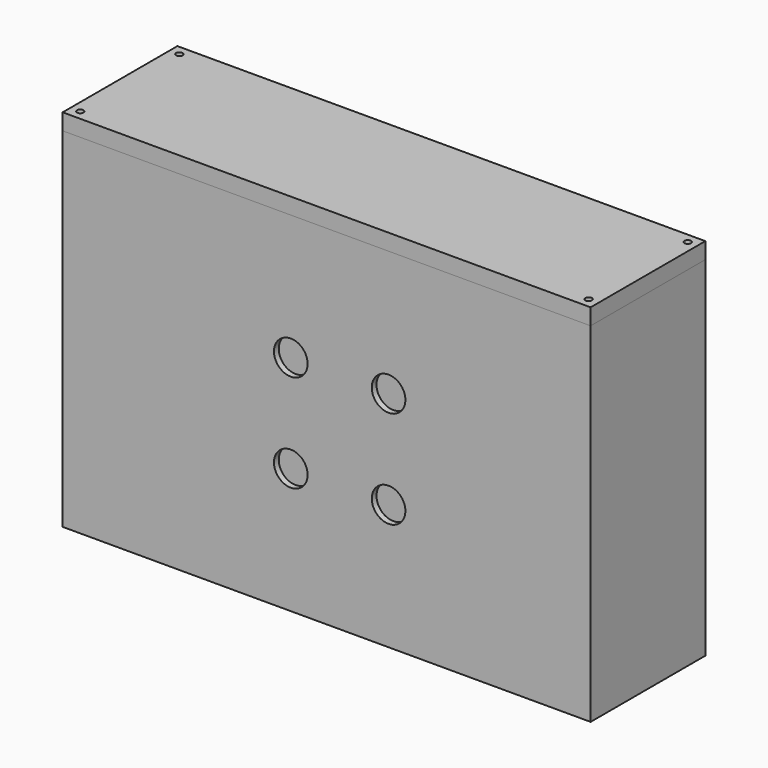
from build123d import *

# Parameters (mm, degrees)
F0_W      = 81
F0_H      = 53.5
F1_DEPTH  = 11
F2_T      = -2.5
F3_W      = 14
F3_H      = 5
F4_DEPTH  = 49.6
F5_R      = 2.5796875
F6_DEPTH  = 25
F8_W      = 81
F8_H      = 22
F9_DEPTH  = 2.5
F11_R     = 0.5
F12_DEPTH = 5
F10_R     = 0.5
F13_DEPTH = 5
F14_R     = 5.159375
F15_DEPTH = 1.5875


# Not quite as in the source:
# - a length typed as a fraction of an inch, garbled in the dataset ("3 / 203.2 mm" for 3/8 in), is restored


with BuildPart() as f1:
    # F0 (on Front) → F1 (new body, symmetric)
    with BuildSketch(Plane.XZ):
        Rectangle(F0_W, F0_H)
    extrude(amount=F1_DEPTH, both=True)

    # F2
    f2_openings = [f1.faces().sort_by_distance(p)[0] for p in [
        (0, 0, 26.75),
    ]]
    offset(amount=F2_T, openings=f2_openings)

    # F3 (on Right) → F4 (cut)
    with BuildSketch(Plane.YZ):
        with Locations((0, -21.75)):
            Rectangle(F3_W, F3_H)
    extrude(amount=-F4_DEPTH, mode=Mode.SUBTRACT)

    # F5 (on Front) → F6 (cut)
    with BuildSketch(Plane.XZ):
        with Locations((-5.5, -7.5)):
            Circle(F5_R)
        with Locations((9.5, -7.5)):
            Circle(F5_R)
        with Locations((9.5, 7.5)):
            Circle(F5_R)
        with Locations((-5.5, 7.5)):
            Circle(F5_R)
    extrude(amount=F6_DEPTH, mode=Mode.SUBTRACT)

    # F11 (on face) → F12 (cut)
    with BuildSketch(Plane.XY.offset(26.75)):
        with Locations((-39, 9.5)):
            Circle(F11_R)
        with Locations((-39, -9.5)):
            Circle(F11_R)
        with Locations((39, -9.5)):
            Circle(F11_R)
        with Locations((39, 9.5)):
            Circle(F11_R)
    extrude(amount=-F12_DEPTH, mode=Mode.SUBTRACT)

    # F14 (on face) → F15 (cut)
    with BuildSketch(Plane(origin=(0, -8.5, 0), x_dir=(-1, 0, 0), z_dir=(0, 1, 0))):
        with Locations((5.5, -7.5)):
            Circle(F14_R)
        with Locations((5.5, 7.5)):
            Circle(F14_R)
        with Locations((-9.5, -7.5)):
            Circle(F14_R)
        with Locations((-9.5, 7.5)):
            Circle(F14_R)
    extrude(amount=-F15_DEPTH, mode=Mode.SUBTRACT)


with BuildPart() as f9:
    # F8 (on offset) → F9 (new body)
    with BuildSketch(Plane.XY.offset(26.75)):
        Rectangle(F8_W, F8_H)
    extrude(amount=F9_DEPTH)

    # F10 (on offset) → F13 (cut, symmetric)
    with BuildSketch(Plane.XY.offset(26.75)):
        with Locations((-39, 9.5)):
            Circle(F10_R)
        with Locations((-39, -9.5)):
            Circle(F10_R)
        with Locations((39, -9.5)):
            Circle(F10_R)
        with Locations((39, 9.5)):
            Circle(F10_R)
    extrude(amount=F13_DEPTH, both=True, mode=Mode.SUBTRACT)


solid = Compound([f1.part, f9.part])
